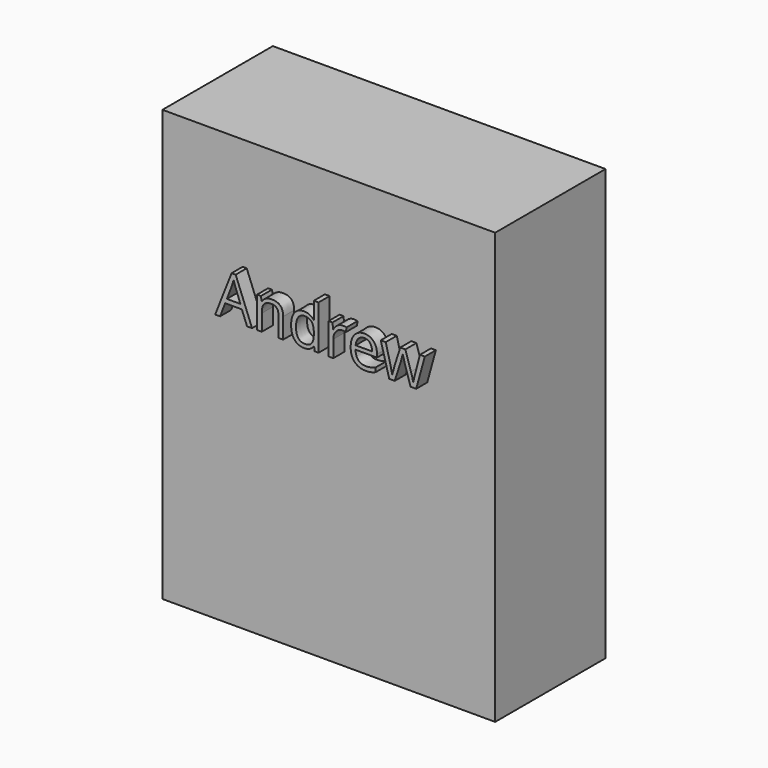
from build123d import *

# Parameters (mm, degrees)
F0_W         = 61.2598918378
F0_H         = 79.2943462729
F1_DEPTH     = 25.4
F2_T         = -2.54
F3_TEXT_SIZE = 10.7347945838
F4_DEPTH     = 27.94


# Not quite as in the source:
# - Text() gives the source's letters only with a copy of the font that has no kerning and outlines rounded to 1/6400 em; it was checked with that copy


with BuildPart() as f1:
    # F0 (on Front) → F1 (new body)
    with BuildSketch(Plane.XZ):
        with Locations((-1.5744362026, -1.5744380653)):
            Rectangle(F0_W, F0_H)
    extrude(amount=F1_DEPTH)

    # F2
    f2_openings = [f1.faces().sort_by_distance(p)[0] for p in [
        (-1.574436, -12.7, -41.221611),
    ]]
    offset(amount=F2_T, openings=f2_openings)

    # F3 (on Front) → F4 (join)
    with BuildSketch(Plane.XZ):
        with Locations((-20.467675291, 9.7328792326)):
            Text('Andrew', F3_TEXT_SIZE, font='Open Sans', text_align=(TextAlign.LEFT, TextAlign.BOTTOM))
    extrude(amount=F4_DEPTH)


solid = f1.part
